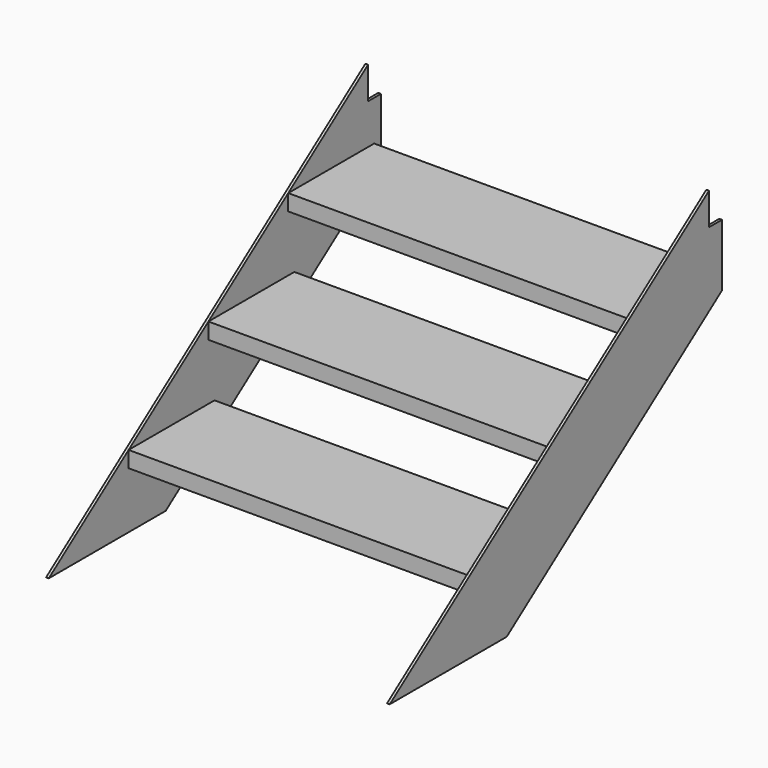
from build123d import *

# Parameters (mm, degrees)
F0_W     = 254
F0_H     = 38.1
F0_W_2   = 235.9806802648
F0_W_3   = 18.0193197352
F1_DEPTH = 6.35
F3_DEPTH = 609.6
F4_R     = 11.1125
F5_DEPTH = 12.7


# Not quite as in the source:
# - a feature names something its author has since deleted; it is built from what else it names


with BuildPart() as f1:
    # F0 (on Right) → F1 (new body)
    with BuildSketch(Plane.YZ):
        Polygon((-943.9227210591, 0), (-598.2182325449, 0), (0, 434.630986972), (0, 476.25), (-235.9806802648, 476.25), (-235.9806802648, 514.35), (-471.9613605296, 342.9), (-707.9420407943, 171.45), align=None)
        with Locations((-580.9420407943, 152.4)):
            Rectangle(F0_W, F0_H, mode=Mode.SUBTRACT)
        with Locations((-344.9613605296, 323.85)):
            Rectangle(F0_W, F0_H, mode=Mode.SUBTRACT)
        Polygon((-235.9806802648, 514.35), (0, 514.35), (0, 609.6), (0, 685.8), align=None)
        with Locations((-344.9613605296, 323.85)):
            Rectangle(F0_W, F0_H)
        with Locations((-580.9420407943, 152.4)):
            Rectangle(F0_W, F0_H)
        with Locations((-117.9903401324, 495.3)):
            Rectangle(F0_W_2, F0_H)
        Polygon((0, 476.25), (0, 434.630986972), (38.1, 462.312257289), (38.1, 609.6), (0, 609.6), (0, 514.35), (18.0193197352, 514.35), (18.0193197352, 476.25), align=None)
        with Locations((9.0096598676, 495.3)):
            Rectangle(F0_W_3, F0_H)
    extrude(amount=-F1_DEPTH)

    # F0 (on Right) → F3 (join)
    with BuildSketch(Plane.YZ):
        with Locations((-344.9613605296, 323.85)):
            Rectangle(F0_W, F0_H)
        with Locations((-580.9420407943, 152.4)):
            Rectangle(F0_W, F0_H)
        with Locations((-117.9903401324, 495.3)):
            Rectangle(F0_W_2, F0_H)
        with Locations((9.0096598676, 495.3)):
            Rectangle(F0_W_3, F0_H)
    extrude(amount=-F3_DEPTH)

    # F4 (on Front) → F5 (cut)
    with BuildSketch(Plane.XZ):
        with Locations((-19.05, 644.525)):
            Circle(F4_R)
    extrude(amount=F5_DEPTH, mode=Mode.SUBTRACT)

    # F6: F1 across plane


with BuildPart() as f1_1:
    add(f1.part)
    add(f1.part.mirror(Plane.YZ.offset(-406.4)))


solid = f1_1.part
